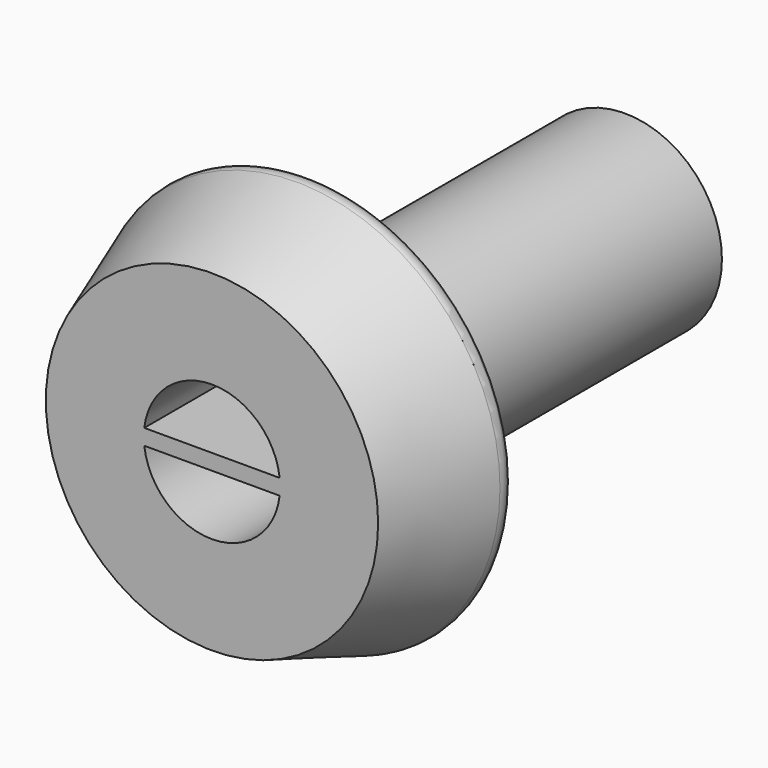
from build123d import *

# Parameters (mm, degrees)
F3_DEPTH = 7.62
F4_R     = 0.635


with BuildPart() as f1:
    # F0 (on Top) → F1 (revolve)
    with BuildSketch(Plane.XY):
        Polygon((3.302, 7.62), (3.302, 4.826), (8.0532941176, 4.826), (10.16, 10.795), (4.699, 10.795), (3.302, 10.795), align=None)
        Polygon((0, 17.145), (0, 12.446), (3.302, 12.446), (3.302, 10.795), (4.699, 10.795), (4.699, 29.845), (2.159, 29.845), (2.159, 17.145), align=None)
    revolve(axis=Axis((0, 23.495, 0), (0, 1, 0)))

    # F2 (on face) → F3 (join)
    with BuildSketch(Plane.XZ.offset(-12.446)):
        with BuildLine():
            ThreePointArc((-3.2799455788, 0.381), (-3.302, 0), (-3.2799455788, -0.381))
            Line((-3.2799455788, -0.381), (3.2799455788, -0.381))
            ThreePointArc((3.2799455788, -0.381), (3.2964817838, -0.1908188916), (3.302, 0))
            ThreePointArc((3.302, 0), (3.2964817838, 0.1908188916), (3.2799455788, 0.381))
            Line((3.2799455788, 0.381), (-3.2799455788, 0.381))
        make_face()
    extrude(amount=F3_DEPTH)

    # F4
    f4_edges = [f1.edges().sort_by_distance(p)[0] for p in [
        (-10.16, 10.795, 0),
    ]]
    fillet(f4_edges, radius=F4_R)


solid = f1.part
